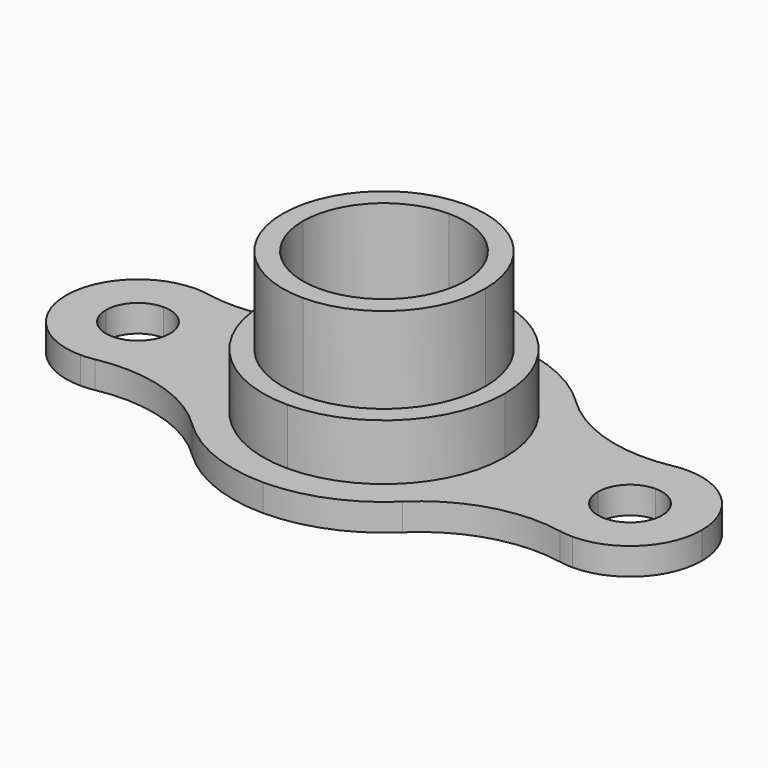
from build123d import *

# Parameters (mm, degrees)
F1_DEPTH = 1.397
F2_DEPTH = 8.7376
F3_DEPTH = 4.2926


# Not quite as in the source:
# - ends of sketch curves that miss each other by under 0.0002 mm in the source are joined


with BuildPart() as f1:
    # F0 (on Top) → F1 (new body)
    with BuildSketch(Plane.XY):
        with BuildLine():
            ThreePointArc((-6.2357, 0), (-4.4093057554, 4.4093057554), (0, 6.2357))
            Line((0, 6.2357), (0, 7.7978))
            ThreePointArc((0, 7.7978), (-2.9283023582, 7.2270831003), (-5.4279628833, 5.5984733435))
            ThreePointArc((-5.4279628833, 5.5984733435), (-8.4727612853, 3.8154532948), (-11.9969014896, 3.6411465506))
            ThreePointArc((-11.9969014896, 3.6411465506), (-12.3468465773, 3.6915461828), (-12.7, 3.7084))
            Line((-12.7, 3.7084), (-12.7, 1.651))
            ThreePointArc((-12.7, 1.651), (-11.5325667043, 1.1674332957), (-11.049, 0))
            Line((-11.049, 0), (-6.2357, 0))
        make_face()
        with BuildLine():
            ThreePointArc((-14.351, 0), (-13.8674332957, 1.1674332957), (-12.7, 1.651))
            Line((-12.7, 1.651), (-12.7, 3.7084))
            ThreePointArc((-12.7, 3.7084), (-15.3222347874, 2.6222347874), (-16.4084, 0))
            Line((-16.4084, 0), (-14.351, 0))
        make_face()
        with BuildLine():
            Line((-12.7, -3.7084), (-12.7, -1.651))
            ThreePointArc((-12.7, -1.651), (-13.8674332957, -1.1674332957), (-14.351, 0))
            Line((-14.351, 0), (-16.4084, 0))
            ThreePointArc((-16.4084, 0), (-15.3222347874, -2.6222347874), (-12.7, -3.7084))
        make_face()
        with BuildLine():
            Line((0, -7.7978), (0, -6.2357))
            ThreePointArc((0, -6.2357), (-4.4093057554, -4.4093057554), (-6.2357, 0))
            Line((-6.2357, 0), (-11.049, 0))
            ThreePointArc((-11.049, 0), (-11.5325667043, -1.1674332957), (-12.7, -1.651))
            Line((-12.7, -1.651), (-12.7, -3.7084))
            ThreePointArc((-12.7, -3.7084), (-12.3468465773, -3.6915461828), (-11.9969031552, -3.6411379247))
            ThreePointArc((-11.9969031552, -3.6411379247), (-8.4727612853, -3.8154532948), (-5.4279673549, -5.5984779556))
            ThreePointArc((-5.4279673549, -5.5984779556), (-2.9283023582, -7.2270831003), (0, -7.7978))
        make_face()
        with BuildLine():
            ThreePointArc((0, -6.2357), (4.4093057554, -4.4093057554), (6.2357, 0))
            Line((6.2357, 0), (5.2324, 0))
            ThreePointArc((5.2324, 0), (3.6998655219, -3.6998655219), (0, -5.2324))
            Line((0, -5.2324), (0, -6.2357))
        make_face()
        with BuildLine():
            ThreePointArc((-6.2357, 0), (-4.4093057554, -4.4093057554), (0, -6.2357))
            Line((0, -6.2357), (0, -5.2324))
            ThreePointArc((0, -5.2324), (-3.6998655219, -3.6998655219), (-5.2324, 0))
            Line((-5.2324, 0), (-6.2357, 0))
        make_face()
        with BuildLine():
            Line((0, 5.2324), (0, 6.2357))
            ThreePointArc((0, 6.2357), (-4.4093057554, 4.4093057554), (-6.2357, 0))
            Line((-6.2357, 0), (-5.2324, 0))
            ThreePointArc((-5.2324, 0), (-3.6998655219, 3.6998655219), (0, 5.2324))
        make_face()
        with BuildLine():
            Line((5.2324, 0), (6.2357, 0))
            ThreePointArc((6.2357, 0), (4.4093057554, 4.4093057554), (0, 6.2357))
            Line((0, 6.2357), (0, 5.2324))
            ThreePointArc((0, 5.2324), (3.6998655219, 3.6998655219), (5.2324, 0))
        make_face()
        with BuildLine():
            ThreePointArc((0, 6.2357), (4.4093057554, 4.4093057554), (6.2357, 0))
            Line((6.2357, 0), (11.049, 0))
            ThreePointArc((11.049, 0), (11.5325667043, 1.1674332957), (12.7, 1.651))
            Line((12.7, 1.651), (12.7, 3.7084))
            ThreePointArc((12.7, 3.7084), (12.3468465773, 3.6915461828), (11.9969031552, 3.6411379247))
            ThreePointArc((11.9969031552, 3.6411379247), (8.4727612853, 3.8154532948), (5.4279673549, 5.5984779556))
            ThreePointArc((5.4279673549, 5.5984779556), (2.9283023582, 7.2270831003), (0, 7.7978))
            Line((0, 7.7978), (0, 6.2357))
        make_face()
        with BuildLine():
            Line((11.049, 0), (6.2357, 0))
            ThreePointArc((6.2357, 0), (4.4093057554, -4.4093057554), (0, -6.2357))
            Line((0, -6.2357), (0, -7.7978))
            ThreePointArc((0, -7.7978), (2.9283023582, -7.2270831003), (5.4279628833, -5.5984733435))
            ThreePointArc((5.4279628833, -5.5984733435), (8.4727612853, -3.8154532948), (11.9969014896, -3.6411465506))
            ThreePointArc((11.9969014896, -3.6411465506), (12.3468465773, -3.6915461828), (12.7, -3.7084))
            Line((12.7, -3.7084), (12.7, -1.651))
            ThreePointArc((12.7, -1.651), (11.5325667043, -1.1674332957), (11.049, 0))
        make_face()
        with BuildLine():
            ThreePointArc((14.351, 0), (13.8674332957, -1.1674332957), (12.7, -1.651))
            Line((12.7, -1.651), (12.7, -3.7084))
            ThreePointArc((12.7, -3.7084), (15.3222347874, -2.6222347874), (16.4084, 0))
            Line((16.4084, 0), (14.351, 0))
        make_face()
        with BuildLine():
            Line((12.7, 3.7084), (12.7, 1.651))
            ThreePointArc((12.7, 1.651), (13.8674332957, 1.1674332957), (14.351, 0))
            Line((14.351, 0), (16.4084, 0))
            ThreePointArc((16.4084, 0), (15.3222347874, 2.6222347874), (12.7, 3.7084))
        make_face()
    extrude(amount=F1_DEPTH)

    # F0 (on Top) → F2 (join)
    with BuildSketch(Plane.XY):
        with BuildLine():
            Line((0, 4.18973), (0, 5.2324))
            ThreePointArc((0, 5.2324), (-3.6998655219, 3.6998655219), (-5.2324, 0))
            Line((-5.2324, 0), (-4.18973, 0))
            ThreePointArc((-4.18973, 0), (-2.9625864943, 2.9625864943), (0, 4.18973))
        make_face()
        with BuildLine():
            Line((4.18973, 0), (5.2324, 0))
            ThreePointArc((5.2324, 0), (3.6998655219, 3.6998655219), (0, 5.2324))
            Line((0, 5.2324), (0, 4.18973))
            ThreePointArc((0, 4.18973), (2.9625864943, 2.9625864943), (4.18973, 0))
        make_face()
        with BuildLine():
            ThreePointArc((0, -5.2324), (3.6998655219, -3.6998655219), (5.2324, 0))
            Line((5.2324, 0), (4.18973, 0))
            ThreePointArc((4.18973, 0), (2.9625864943, -2.9625864943), (0, -4.18973))
            Line((0, -4.18973), (0, -5.2324))
        make_face()
        with BuildLine():
            ThreePointArc((-5.2324, 0), (-3.6998655219, -3.6998655219), (0, -5.2324))
            Line((0, -5.2324), (0, -4.18973))
            ThreePointArc((0, -4.18973), (-2.9625864943, -2.9625864943), (-4.18973, 0))
            Line((-4.18973, 0), (-5.2324, 0))
        make_face()
    extrude(amount=F2_DEPTH)

    # F0 (on Top) → F3 (join)
    with BuildSketch(Plane.XY):
        with BuildLine():
            ThreePointArc((-6.2357, 0), (-4.4093057554, -4.4093057554), (0, -6.2357))
            Line((0, -6.2357), (0, -5.2324))
            ThreePointArc((0, -5.2324), (-3.6998655219, -3.6998655219), (-5.2324, 0))
            Line((-5.2324, 0), (-6.2357, 0))
        make_face()
        with BuildLine():
            ThreePointArc((0, -6.2357), (4.4093057554, -4.4093057554), (6.2357, 0))
            Line((6.2357, 0), (5.2324, 0))
            ThreePointArc((5.2324, 0), (3.6998655219, -3.6998655219), (0, -5.2324))
            Line((0, -5.2324), (0, -6.2357))
        make_face()
        with BuildLine():
            Line((5.2324, 0), (6.2357, 0))
            ThreePointArc((6.2357, 0), (4.4093057554, 4.4093057554), (0, 6.2357))
            Line((0, 6.2357), (0, 5.2324))
            ThreePointArc((0, 5.2324), (3.6998655219, 3.6998655219), (5.2324, 0))
        make_face()
        with BuildLine():
            Line((0, 5.2324), (0, 6.2357))
            ThreePointArc((0, 6.2357), (-4.4093057554, 4.4093057554), (-6.2357, 0))
            Line((-6.2357, 0), (-5.2324, 0))
            ThreePointArc((-5.2324, 0), (-3.6998655219, 3.6998655219), (0, 5.2324))
        make_face()
    extrude(amount=F3_DEPTH)


solid = f1.part
